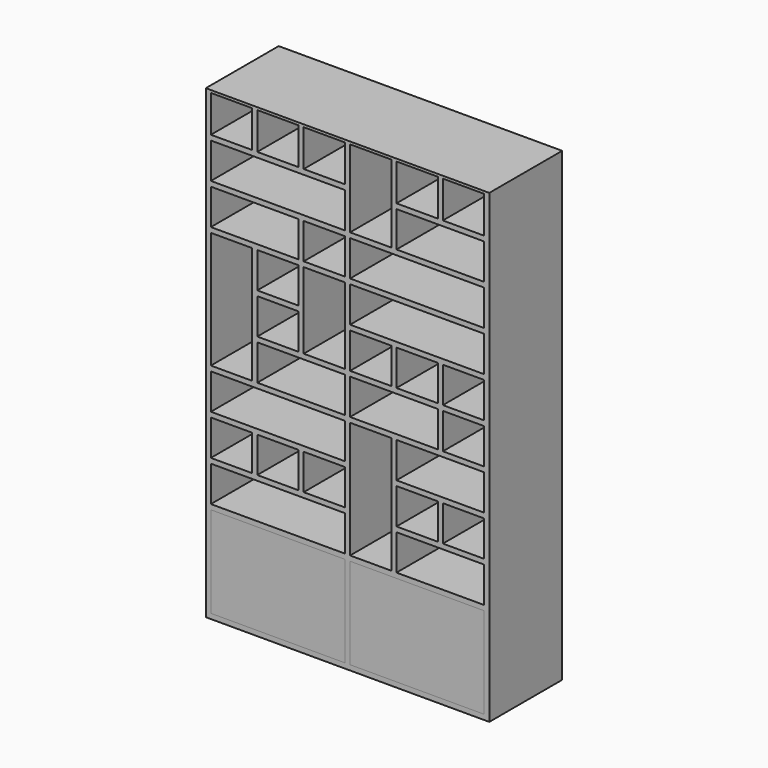
from build123d import *

# Parameters (mm, degrees)
F0_W     = 1400
F0_H     = 2300
F1_DEPTH = 450
F2_W     = 204.1666666667
F2_H     = 181.9444444444
F2_H_2   = 382.6388888889
F2_W_2   = 662.5
F2_H_3   = 175.6944444444
F2_W_3   = 433.3333333333
F2_H_4   = 577.0833333333
F2_H_5   = 376.3888888889
F2_H_6   = 450
F3_DEPTH = 425
F4_DEPTH = 425
F5_T     = -15
F5_2_T   = -15


with BuildPart() as f1:
    # F0 (on Front) → F1 (new body)
    with BuildSketch(Plane.XZ):
        with Locations((0, 1150)):
            Rectangle(F0_W, F0_H)
    extrude(amount=F1_DEPTH)

    # F2 (on face) → F3 (cut, through all)
    with BuildSketch(Plane.XZ.offset(450)):
        with Locations((-572.9166666667, 2196.5277777778)):
            Rectangle(F2_W, F2_H)
        with Locations((-343.75, 2196.5277777778)):
            Rectangle(F2_W, F2_H)
        with Locations((-114.5833333333, 2196.5277777778)):
            Rectangle(F2_W, F2_H)
        with Locations((114.5833333333, 2096.1805555556)):
            Rectangle(F2_W, F2_H_2)
        with Locations((343.75, 2196.5277777778)):
            Rectangle(F2_W, F2_H)
        with Locations((572.9166666667, 2196.5277777778)):
            Rectangle(F2_W, F2_H)
        with Locations((-343.75, 1992.7083333333)):
            Rectangle(F2_W_2, F2_H_3)
        with Locations((458.3333333333, 1992.7083333333)):
            Rectangle(F2_W_3, F2_H_3)
        with Locations((-458.3333333333, 1792.0138888889)):
            Rectangle(F2_W_3, F2_H_3)
        with Locations((-114.5833333333, 1792.0138888889)):
            Rectangle(F2_W, F2_H_3)
        with Locations((343.75, 1792.0138888889)):
            Rectangle(F2_W_2, F2_H_3)
        with Locations((-572.9166666667, 1390.625)):
            Rectangle(F2_W, F2_H_4)
        with Locations((-343.75, 1591.3194444444)):
            Rectangle(F2_W, F2_H_3)
        with Locations((-343.75, 1390.625)):
            Rectangle(F2_W, F2_H_3)
        with Locations((-229.1666666667, 1189.9305555556)):
            Rectangle(F2_W_3, F2_H_3)
        with Locations((-114.5833333333, 1490.9722222222)):
            Rectangle(F2_W, F2_H_5)
        with Locations((343.75, 1591.3194444444)):
            Rectangle(F2_W_2, F2_H_3)
        with Locations((114.5833333333, 1390.625)):
            Rectangle(F2_W, F2_H_3)
        with Locations((343.75, 1390.625)):
            Rectangle(F2_W, F2_H_3)
        with Locations((572.9166666667, 1390.625)):
            Rectangle(F2_W, F2_H_3)
        with Locations((229.1666666667, 1189.9305555556)):
            Rectangle(F2_W_3, F2_H_3)
        with Locations((572.9166666667, 1189.9305555556)):
            Rectangle(F2_W, F2_H_3)
        with Locations((-343.75, 989.2361111111)):
            Rectangle(F2_W_2, F2_H_3)
        with Locations((-572.9166666667, 788.5416666667)):
            Rectangle(F2_W, F2_H_3)
        with Locations((-343.75, 788.5416666667)):
            Rectangle(F2_W, F2_H_3)
        with Locations((-114.5833333333, 788.5416666667)):
            Rectangle(F2_W, F2_H_3)
        with Locations((-343.75, 587.8472222222)):
            Rectangle(F2_W_2, F2_H_3)
        with Locations((114.5833333333, 788.5416666667)):
            Rectangle(F2_W, F2_H_4)
        with Locations((458.3333333333, 989.2361111111)):
            Rectangle(F2_W_3, F2_H_3)
        with Locations((343.75, 788.5416666667)):
            Rectangle(F2_W, F2_H_3)
        with Locations((572.9166666667, 788.5416666667)):
            Rectangle(F2_W, F2_H_3)
        with Locations((458.3333333333, 587.8472222222)):
            Rectangle(F2_W_3, F2_H_3)
        with Locations((-343.75, 250)):
            Rectangle(F2_W_2, F2_H_6)
        with Locations((343.75, 250)):
            Rectangle(F2_W_2, F2_H_6)
    extrude(amount=-F3_DEPTH, mode=Mode.SUBTRACT)


with BuildPart() as f4:
    # F2 (on face) → F4 (new body, through all)
    with BuildSketch(Plane.XZ.offset(450)):
        with Locations((-343.75, 250)):
            Rectangle(F2_W_2, F2_H_6)
    extrude(amount=-F4_DEPTH)

    # F5
    f5_openings = [f4.faces().sort_by_distance(p)[0] for p in [
        (-343.75, -237.5, 475),
    ]]
    offset(amount=F5_T, openings=f5_openings)


with BuildPart() as f4b:
    # F2 (on face) → F4, piece 2 (new body, through all)
    with BuildSketch(Plane.XZ.offset(450)):
        with Locations((343.75, 250)):
            Rectangle(F2_W_2, F2_H_6)
    extrude(amount=-F4_DEPTH)

    # F5#2
    f5_2_openings = [f4b.faces().sort_by_distance(p)[0] for p in [
        (343.75, -237.5, 475),
    ]]
    offset(amount=F5_2_T, openings=f5_2_openings)


solid = Compound([f1.part, f4.part, f4b.part])
